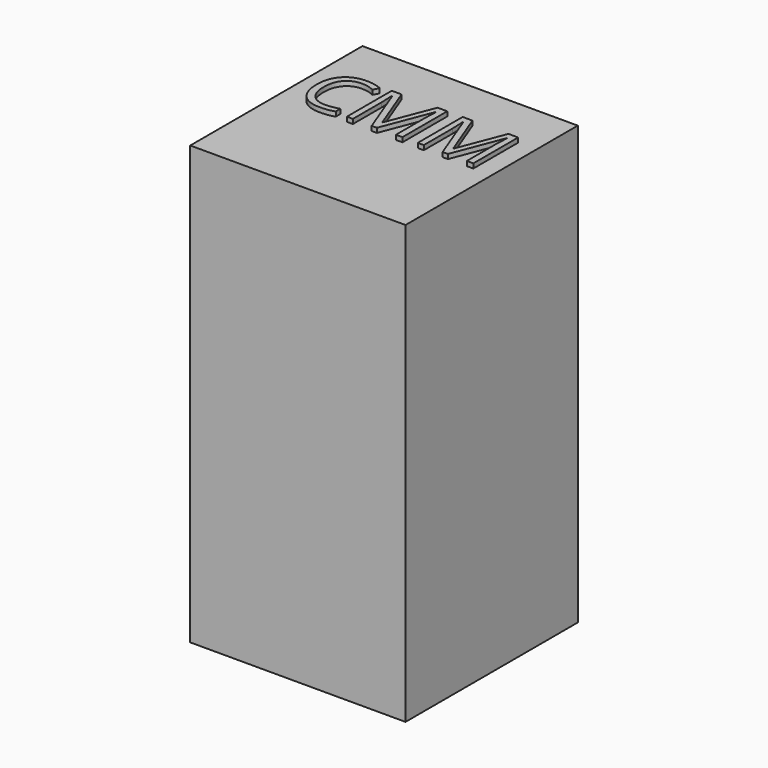
from build123d import *

# Parameters (mm, degrees)
F0_W         = 1200
F0_H         = 1200
F1_DEPTH     = 2438.4
F2_TEXT_SIZE = 437.863667806
F3_DEPTH     = 25.4


# Not quite as in the source:
# - Text() gives the source's letters only with a copy of the font that has no kerning and outlines rounded to 1/6400 em; it was checked with that copy


with BuildPart() as f1:
    # F0 (on Top) → F1 (new body)
    with BuildSketch(Plane.XY):
        Rectangle(F0_W, F0_H)
    extrude(amount=F1_DEPTH)

    # F2 (on face) → F3 (join)
    with BuildSketch(Plane.XY.offset(2438.4)):
        with Locations((-526.2573957443, 0)):
            Text('CMM', F2_TEXT_SIZE, font='Open Sans', text_align=(TextAlign.LEFT, TextAlign.BOTTOM))
    extrude(amount=F3_DEPTH)


solid = f1.part
